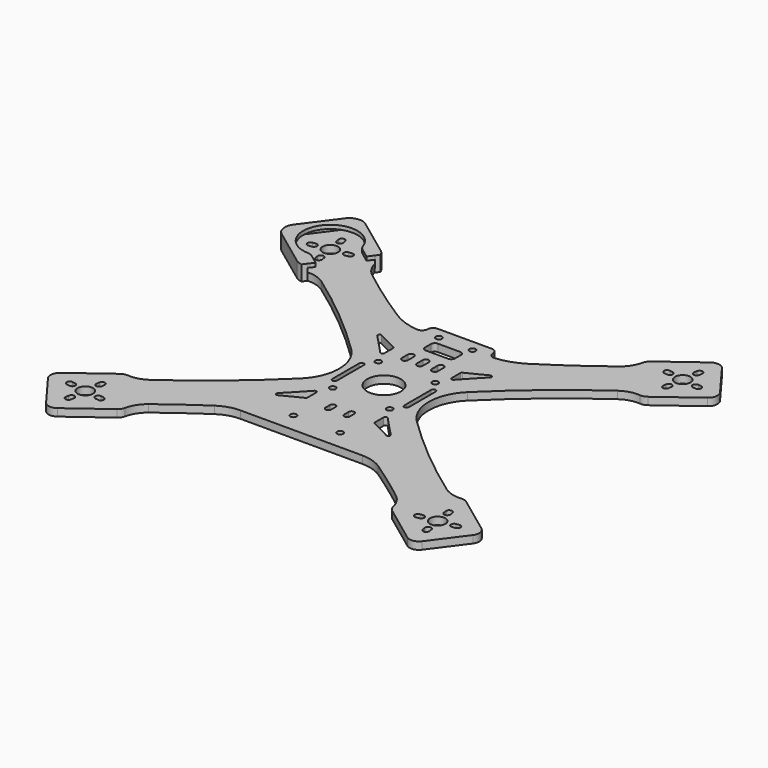
from build123d import *

# Parameters (mm, degrees)
F0_R      = 4.125
F0_R_2    = 1.625
F1_DEPTH  = 4
F3_DEPTH  = 25
F5_DEPTH  = 25
F6_R      = 9
F7_DEPTH  = 25
F8_R      = 3
F10_DEPTH = 25
F12_DEPTH = 8.1
F13_START = 2
F13_DEPTH = 4.1
F15_START = 5
F15_DEPTH = 5
F16_R     = 13
F17_DEPTH = 25


with BuildPart() as f1:
    # F0 (on Top) → F1 (new body)
    with BuildSketch(Plane.XY):
        with BuildLine():
            Line((-100.6321728581, 100.3756166522), (-113.7425143861, 82.7087282725))
            ThreePointArc((-113.7425143861, 82.7087282725), (-114.6734006575, 78.9968403849), (-112.7069355562, 75.7139032935))
            Line((-112.7069355562, 75.7139032935), (-92.6704812737, 60.8451412903))
            ThreePointArc((-92.6704812737, 60.8451412903), (-91.0578143808, 60.0508285833), (-89.2684477777, 59.8782182027))
            ThreePointArc((-89.2684477777, 59.8782182027), (-84.0566311488, 59.4038937484), (-79.3249672671, 57.1679659385))
            ThreePointArc((-79.3249672671, 57.1679659385), (-54.451545195, 38.0227925286), (-31.1542479846, 16.9880419203))
            ThreePointArc((-31.1542479846, 16.9880419203), (-24, 0), (-31.1542479846, -16.9880419203))
            ThreePointArc((-31.1542479846, -16.9880419203), (-54.451545195, -38.0227925286), (-79.3249672671, -57.1679659385))
            ThreePointArc((-79.3249672671, -57.1679659385), (-84.0566311488, -59.4038937484), (-89.2684477777, -59.8782182027))
            ThreePointArc((-89.2684477777, -59.8782182027), (-91.0578143808, -60.0508285833), (-92.6704812737, -60.8451412903))
            Line((-92.6704812737, -60.8451412903), (-112.7069355562, -75.7139032935))
            ThreePointArc((-112.7069355562, -75.7139032935), (-114.6734006575, -78.9968403849), (-113.7425143861, -82.7087282725))
            Line((-113.7425143861, -82.7087282725), (-100.6321728581, -100.3756166522))
            ThreePointArc((-100.6321728581, -100.3756166522), (-97.3492357667, -102.3420817535), (-93.6373478791, -101.4111954821))
            Line((-93.6373478791, -101.4111954821), (-73.6008935965, -86.5424334789))
            ThreePointArc((-73.6008935965, -86.5424334789), (-72.3733879407, -85.229095347), (-71.6897171476, -83.5665005586))
            ThreePointArc((-71.6897171476, -83.5665005586), (-69.7256278453, -78.7156893405), (-66.2146257391, -74.8348543181))
            ThreePointArc((-66.2146257391, -74.8348543181), (-55.1443985805, -66.5447330976), (-43.7944655315, -58.6418817782))
            ThreePointArc((-43.7944655315, -58.6418817782), (-38.4752742537, -56.1167519167), (-32.651287837, -55.25))
            Line((-32.651287837, -55.25), (32.651287837, -55.25))
            ThreePointArc((32.651287837, -55.25), (38.4752742537, -56.1167519167), (43.7944655315, -58.6418817782))
            ThreePointArc((43.7944655315, -58.6418817782), (55.1443985805, -66.5447330976), (66.2146257391, -74.8348543181))
            ThreePointArc((66.2146257391, -74.8348543181), (69.7256278453, -78.7156893405), (71.6897171476, -83.5665005586))
            ThreePointArc((71.6897171476, -83.5665005586), (72.3733879407, -85.229095347), (73.6008935965, -86.5424334789))
            Line((73.6008935965, -86.5424334789), (93.6373478791, -101.4111954821))
            ThreePointArc((93.6373478791, -101.4111954821), (97.3492357667, -102.3420817535), (100.6321728581, -100.3756166522))
            Line((100.6321728581, -100.3756166522), (113.7425143861, -82.7087282725))
            ThreePointArc((113.7425143861, -82.7087282725), (114.6734006575, -78.9968403849), (112.7069355562, -75.7139032935))
            Line((112.7069355562, -75.7139032935), (92.6704812737, -60.8451412903))
            ThreePointArc((92.6704812737, -60.8451412903), (91.0578143808, -60.0508285833), (89.2684477777, -59.8782182027))
            ThreePointArc((89.2684477777, -59.8782182027), (84.0566311488, -59.4038937484), (79.3249672671, -57.1679659385))
            ThreePointArc((79.3249672671, -57.1679659385), (54.451545195, -38.0227925286), (31.1542479846, -16.9880419203))
            ThreePointArc((31.1542479846, -16.9880419203), (24, 0), (31.1542479846, 16.9880419203))
            ThreePointArc((31.1542479846, 16.9880419203), (54.451545195, 38.0227925286), (79.3249672671, 57.1679659385))
            ThreePointArc((79.3249672671, 57.1679659385), (84.0566311488, 59.4038937484), (89.2684477777, 59.8782182027))
            ThreePointArc((89.2684477777, 59.8782182027), (91.0578143808, 60.0508285833), (92.6704812737, 60.8451412903))
            Line((92.6704812737, 60.8451412903), (112.7069355562, 75.7139032935))
            ThreePointArc((112.7069355562, 75.7139032935), (114.6734006575, 78.9968403849), (113.7425143861, 82.7087282725))
            Line((113.7425143861, 82.7087282725), (100.6321728581, 100.3756166522))
            ThreePointArc((100.6321728581, 100.3756166522), (97.3492357667, 102.3420817535), (93.6373478791, 101.4111954821))
            Line((93.6373478791, 101.4111954821), (73.6008935965, 86.5424334789))
            ThreePointArc((73.6008935965, 86.5424334789), (72.3733879407, 85.229095347), (71.6897171476, 83.5665005586))
            ThreePointArc((71.6897171476, 83.5665005586), (69.7256278453, 78.7156893405), (66.2146257391, 74.8348543181))
            ThreePointArc((66.2146257391, 74.8348543181), (50.8276984936, 63.4702586312), (34.9155456792, 52.8535285321))
            ThreePointArc((34.9155456792, 52.8535285321), (28.1194648937, 49.62008029), (20.7483484329, 48.1006910376))
            ThreePointArc((20.7483484329, 48.1006910376), (18.4683806088, 48.8830147391), (17.5, 51.090393875))
            Line((17.5, 51.090393875), (17.5, 54))
            Line((17.5, 54), (0, 54))
            Line((0, 54), (-17.5, 54))
            Line((-17.5, 54), (-17.5, 51.090393875))
            ThreePointArc((-17.5, 51.090393875), (-18.4683806088, 48.8830147391), (-20.7483484329, 48.1006910376))
            ThreePointArc((-20.7483484329, 48.1006910376), (-28.1194648937, 49.62008029), (-34.9155456792, 52.8535285321))
            ThreePointArc((-34.9155456792, 52.8535285321), (-50.8276984936, 63.4702586312), (-66.2146257391, 74.8348543181))
            ThreePointArc((-66.2146257391, 74.8348543181), (-69.7256278453, 78.7156893405), (-71.6897171476, 83.5665005586))
            ThreePointArc((-71.6897171476, 83.5665005586), (-72.3733879407, 85.229095347), (-73.6008935965, 86.5424334789))
            Line((-73.6008935965, 86.5424334789), (-93.6373478791, 101.4111954821))
            ThreePointArc((-93.6373478791, 101.4111954821), (-97.3492357667, 102.3420817535), (-100.6321728581, 100.3756166522))
        make_face()
        with Locations((-94.3386975278, -82.0073786238)):
            Circle(F0_R, mode=Mode.SUBTRACT)
        with Locations((-12.5, -45)):
            Circle(F0_R_2, mode=Mode.SUBTRACT)
        with Locations((-15.25, -15.25)):
            Circle(F0_R_2, mode=Mode.SUBTRACT)
        with Locations((94.3386975278, -82.0073786238)):
            Circle(F0_R, mode=Mode.SUBTRACT)
        with Locations((12.5, -45)):
            Circle(F0_R_2, mode=Mode.SUBTRACT)
        with Locations((15.25, -15.25)):
            Circle(F0_R_2, mode=Mode.SUBTRACT)
        with BuildLine():
            Line((-20.5, -9), (-20.5, 9))
            ThreePointArc((-20.5, 9), (-19.25, 10.25), (-18, 9))
            Line((-18, 9), (-18, -9))
            ThreePointArc((-18, -9), (-19.25, -10.25), (-20.5, -9))
        make_face(mode=Mode.SUBTRACT)
        with Locations((-15.25, 15.25)):
            Circle(F0_R_2, mode=Mode.SUBTRACT)
        with Locations((-9, 48)):
            Circle(F0_R_2, mode=Mode.SUBTRACT)
        with Locations((-94.3386975278, 82.0073786238)):
            Circle(F0_R, mode=Mode.SUBTRACT)
        with BuildLine():
            ThreePointArc((18, 9), (19.25, 10.25), (20.5, 9))
            Line((20.5, 9), (20.5, -9))
            ThreePointArc((20.5, -9), (19.25, -10.25), (18, -9))
            Line((18, -9), (18, 9))
        make_face(mode=Mode.SUBTRACT)
        with Locations((15.25, 15.25)):
            Circle(F0_R_2, mode=Mode.SUBTRACT)
        with Locations((9, 48)):
            Circle(F0_R_2, mode=Mode.SUBTRACT)
        with Locations((94.3386975278, 82.0073786238)):
            Circle(F0_R, mode=Mode.SUBTRACT)
    extrude(amount=F1_DEPTH)

    # F2 (on face) → F3 (cut)
    with BuildSketch(Plane.XY.offset(4)):
        with BuildLine():
            ThreePointArc((-97.1104772378, 89.6336727592), (-95.2650125164, 88.2641801663), (-93.8955199235, 90.1096448877))
            Line((-93.8955199235, 90.1096448877), (-94.1298446637, 91.692393104))
            ThreePointArc((-94.1298446637, 91.692393104), (-95.9753093851, 93.0618856969), (-97.344801978, 91.2164209755))
            Line((-97.344801978, 91.2164209755), (-97.1104772378, 89.6336727592))
        make_face()
        with BuildLine():
            ThreePointArc((-101.9649916632, 79.2355989138), (-100.5954990703, 81.0810636353), (-102.4409637917, 82.4505562282))
            Line((-102.4409637917, 82.4505562282), (-104.023712008, 82.216231488))
            ThreePointArc((-104.023712008, 82.216231488), (-105.3932046009, 80.3707667666), (-103.5477398795, 79.0012741737))
            Line((-103.5477398795, 79.0012741737), (-101.9649916632, 79.2355989138))
        make_face()
        with BuildLine():
            ThreePointArc((-91.5669178179, 74.3810844884), (-93.4123825393, 75.7505770813), (-94.7818751322, 73.9051123599))
            Line((-94.7818751322, 73.9051123599), (-94.547550392, 72.3223641436))
            ThreePointArc((-94.547550392, 72.3223641436), (-92.7020856706, 70.9528715507), (-91.3325930777, 72.7983362721))
            Line((-91.3325930777, 72.7983362721), (-91.5669178179, 74.3810844884))
        make_face()
        with BuildLine():
            ThreePointArc((-86.7124033925, 84.7791583338), (-88.0818959854, 82.9336936124), (-86.236431264, 81.5642010195))
            Line((-86.236431264, 81.5642010195), (-84.6536830477, 81.7985257596))
            ThreePointArc((-84.6536830477, 81.7985257596), (-83.2841904548, 83.6439904811), (-85.1296551762, 85.013483074))
            Line((-85.1296551762, 85.013483074), (-86.7124033925, 84.7791583338))
        make_face()
        with BuildLine():
            Line((94.1298446637, 91.692393104), (93.8955199235, 90.1096448877))
            ThreePointArc((93.8955199235, 90.1096448877), (95.2650125164, 88.2641801663), (97.1104772378, 89.6336727592))
            Line((97.1104772378, 89.6336727592), (97.344801978, 91.2164209755))
            ThreePointArc((97.344801978, 91.2164209755), (95.9753093851, 93.0618856969), (94.1298446637, 91.692393104))
        make_face()
        with BuildLine():
            Line((104.023712008, 82.216231488), (102.4409637917, 82.4505562282))
            ThreePointArc((102.4409637917, 82.4505562282), (100.5954990703, 81.0810636353), (101.9649916632, 79.2355989138))
            Line((101.9649916632, 79.2355989138), (103.5477398795, 79.0012741737))
            ThreePointArc((103.5477398795, 79.0012741737), (105.3932046009, 80.3707667666), (104.023712008, 82.216231488))
        make_face()
        with BuildLine():
            ThreePointArc((86.236431264, 81.5642010195), (88.0818959854, 82.9336936124), (86.7124033925, 84.7791583338))
            Line((86.7124033925, 84.7791583338), (85.1296551762, 85.013483074))
            ThreePointArc((85.1296551762, 85.013483074), (83.2841904548, 83.6439904811), (84.6536830477, 81.7985257596))
            Line((84.6536830477, 81.7985257596), (86.236431264, 81.5642010195))
        make_face()
        with BuildLine():
            Line((94.547550392, 72.3223641436), (94.7818751322, 73.9051123599))
            ThreePointArc((94.7818751322, 73.9051123599), (93.4123825393, 75.7505770813), (91.5669178179, 74.3810844884))
            Line((91.5669178179, 74.3810844884), (91.3325930777, 72.7983362721))
            ThreePointArc((91.3325930777, 72.7983362721), (92.7020856706, 70.9528715507), (94.547550392, 72.3223641436))
        make_face()
        with BuildLine():
            Line((-94.1298446637, -91.692393104), (-93.8955199235, -90.1096448877))
            ThreePointArc((-93.8955199235, -90.1096448877), (-95.2650125164, -88.2641801663), (-97.1104772378, -89.6336727592))
            Line((-97.1104772378, -89.6336727592), (-97.344801978, -91.2164209755))
            ThreePointArc((-97.344801978, -91.2164209755), (-95.9753093851, -93.0618856969), (-94.1298446637, -91.692393104))
        make_face()
        with BuildLine():
            Line((-104.023712008, -82.216231488), (-102.4409637917, -82.4505562282))
            ThreePointArc((-102.4409637917, -82.4505562282), (-100.5954990703, -81.0810636353), (-101.9649916632, -79.2355989138))
            Line((-101.9649916632, -79.2355989138), (-103.5477398795, -79.0012741737))
            ThreePointArc((-103.5477398795, -79.0012741737), (-105.3932046009, -80.3707667666), (-104.023712008, -82.216231488))
        make_face()
        with BuildLine():
            ThreePointArc((86.7124033925, -84.7791583338), (88.0818959854, -82.9336936124), (86.236431264, -81.5642010195))
            Line((86.236431264, -81.5642010195), (84.6536830477, -81.7985257596))
            ThreePointArc((84.6536830477, -81.7985257596), (83.2841904548, -83.6439904811), (85.1296551762, -85.013483074))
            Line((85.1296551762, -85.013483074), (86.7124033925, -84.7791583338))
        make_face()
        with BuildLine():
            Line((97.344801978, -91.2164209755), (97.1104772378, -89.6336727592))
            ThreePointArc((97.1104772378, -89.6336727592), (95.2650125164, -88.2641801663), (93.8955199235, -90.1096448877))
            Line((93.8955199235, -90.1096448877), (94.1298446637, -91.692393104))
            ThreePointArc((94.1298446637, -91.692393104), (95.9753093851, -93.0618856969), (97.344801978, -91.2164209755))
        make_face()
        with BuildLine():
            Line((103.5477398795, -79.0012741737), (101.9649916632, -79.2355989138))
            ThreePointArc((101.9649916632, -79.2355989138), (100.5954990703, -81.0810636353), (102.4409637917, -82.4505562282))
            Line((102.4409637917, -82.4505562282), (104.023712008, -82.216231488))
            ThreePointArc((104.023712008, -82.216231488), (105.3932046009, -80.3707667666), (103.5477398795, -79.0012741737))
        make_face()
        with BuildLine():
            Line((91.3325930777, -72.7983362721), (91.5669178179, -74.3810844884))
            ThreePointArc((91.5669178179, -74.3810844884), (93.4123825393, -75.7505770813), (94.7818751322, -73.9051123599))
            Line((94.7818751322, -73.9051123599), (94.547550392, -72.3223641436))
            ThreePointArc((94.547550392, -72.3223641436), (92.7020856706, -70.9528715507), (91.3325930777, -72.7983362721))
        make_face()
        with BuildLine():
            ThreePointArc((-94.7818751322, -73.9051123599), (-93.4123825393, -75.7505770813), (-91.5669178179, -74.3810844884))
            Line((-91.5669178179, -74.3810844884), (-91.3325930777, -72.7983362721))
            ThreePointArc((-91.3325930777, -72.7983362721), (-92.7020856706, -70.9528715507), (-94.547550392, -72.3223641436))
            Line((-94.547550392, -72.3223641436), (-94.7818751322, -73.9051123599))
        make_face()
        with BuildLine():
            Line((-86.7124033925, -84.7791583338), (-85.1296551762, -85.013483074))
            ThreePointArc((-85.1296551762, -85.013483074), (-83.2841904548, -83.6439904811), (-84.6536830477, -81.7985257596))
            Line((-84.6536830477, -81.7985257596), (-86.236431264, -81.5642010195))
            ThreePointArc((-86.236431264, -81.5642010195), (-88.0818959854, -82.9336936124), (-86.7124033925, -84.7791583338))
        make_face()
    extrude(amount=-F3_DEPTH, mode=Mode.SUBTRACT)

    # F4 (on face) → F5 (cut)
    with BuildSketch(Plane.XY.offset(4)):
        with BuildLine():
            ThreePointArc((-6.375, 28), (-8, 29.625), (-9.625, 28))
            Line((-9.625, 28), (-9.625, 24))
            ThreePointArc((-9.625, 24), (-8, 22.375), (-6.375, 24))
            Line((-6.375, 24), (-6.375, 28))
        make_face()
        with BuildLine():
            ThreePointArc((1.625, 28), (0, 29.625), (-1.625, 28))
            Line((-1.625, 28), (-1.625, 24))
            ThreePointArc((-1.625, 24), (0, 22.375), (1.625, 24))
            Line((1.625, 24), (1.625, 28))
        make_face()
        with BuildLine():
            ThreePointArc((9.625, 28), (8, 29.625), (6.375, 28))
            Line((6.375, 28), (6.375, 24))
            ThreePointArc((6.375, 24), (8, 22.375), (9.625, 24))
            Line((9.625, 24), (9.625, 28))
        make_face()
    extrude(amount=-F5_DEPTH, mode=Mode.SUBTRACT)

    # F6 (on face) → F7 (cut)
    with BuildSketch(Plane.XY.offset(4)):
        with BuildLine():
            Line((6, 43.5), (-6, 43.5))
            ThreePointArc((-6, 43.5), (-7.4142135624, 42.9142135624), (-8, 41.5))
            Line((-8, 41.5), (-8, 37.5))
            ThreePointArc((-8, 37.5), (-7.4142135624, 36.0857864376), (-6, 35.5))
            Line((-6, 35.5), (6, 35.5))
            ThreePointArc((6, 35.5), (7.4142135624, 36.0857864376), (8, 37.5))
            Line((8, 37.5), (8, 41.5))
            ThreePointArc((8, 41.5), (7.4142135624, 42.9142135624), (6, 43.5))
        make_face()
        with BuildLine():
            ThreePointArc((-3.5, -28), (-5, -26.5), (-6.5, -28))
            Line((-6.5, -28), (-6.5, -31))
            ThreePointArc((-6.5, -31), (-5, -32.5), (-3.5, -31))
            Line((-3.5, -31), (-3.5, -28))
        make_face()
        with BuildLine():
            ThreePointArc((6.5, -28), (5, -26.5), (3.5, -28))
            Line((3.5, -28), (3.5, -31))
            ThreePointArc((3.5, -31), (5, -32.5), (6.5, -31))
            Line((6.5, -31), (6.5, -28))
        make_face()
        Circle(F6_R)
    extrude(amount=-F7_DEPTH, mode=Mode.SUBTRACT)

    # F8
    f8_edges = [f1.edges().sort_by_distance(p)[0] for p in [
        (-17.5, 54, 2),
        (17.5, 54, 2),
    ]]
    fillet(f8_edges, radius=F8_R)

    # F9 (on face) → F10 (cut)
    with BuildSketch(Plane.XY.offset(4)):
        with BuildLine():
            ThreePointArc((-18.5615734392, 29.4784741395), (-23.8228134976, 32.0929109704), (-29.0451265181, 34.7842626031))
            ThreePointArc((-29.0451265181, 34.7842626031), (-30.3127764029, 34.494671544), (-30.2226462445, 33.1974916156))
            ThreePointArc((-30.2226462445, 33.1974916156), (-24.9281613816, 27.7115010311), (-19.7390931656, 22.1256945802))
            ThreePointArc((-19.7390931656, 22.1256945802), (-18.6388166433, 21.8668029796), (-18, 22.7992977961))
            Line((-18, 22.7992977961), (-18, 28.5797071226))
            ThreePointArc((-18, 28.5797071226), (-18.1519355682, 29.1096002435), (-18.5615734392, 29.4784741395))
        make_face()
        with BuildLine():
            ThreePointArc((18.5615734392, 29.4784741395), (18.1519355682, 29.1096002435), (18, 28.5797071226))
            Line((18, 28.5797071226), (18, 22.7992977961))
            ThreePointArc((18, 22.7992977961), (18.6388166433, 21.8668029796), (19.7390931656, 22.1256945802))
            ThreePointArc((19.7390931656, 22.1256945802), (24.9281613816, 27.7115010311), (30.2226462445, 33.1974916156))
            ThreePointArc((30.2226462445, 33.1974916156), (30.3127764029, 34.494671544), (29.0451265181, 34.7842626031))
            ThreePointArc((29.0451265181, 34.7842626031), (23.8228134976, 32.0929109704), (18.5615734392, 29.4784741395))
        make_face()
        with BuildLine():
            Line((18, -22.7992977961), (18, -28.5797071226))
            ThreePointArc((18, -28.5797071226), (18.1519355682, -29.1096002435), (18.5615734392, -29.4784741395))
            ThreePointArc((18.5615734392, -29.4784741395), (23.8228134976, -32.0929109704), (29.0451265181, -34.7842626031))
            ThreePointArc((29.0451265181, -34.7842626031), (30.3127764029, -34.494671544), (30.2226462445, -33.1974916156))
            ThreePointArc((30.2226462445, -33.1974916156), (24.9281613816, -27.7115010311), (19.7390931656, -22.1256945802))
            ThreePointArc((19.7390931656, -22.1256945802), (18.6388166433, -21.8668029796), (18, -22.7992977961))
        make_face()
        with BuildLine():
            ThreePointArc((-18.5615734392, -29.4784741395), (-18.1519355682, -29.1096002435), (-18, -28.5797071226))
            Line((-18, -28.5797071226), (-18, -22.7992977961))
            ThreePointArc((-18, -22.7992977961), (-18.6388166433, -21.8668029796), (-19.7390931656, -22.1256945802))
            ThreePointArc((-19.7390931656, -22.1256945802), (-24.9281613816, -27.7115010311), (-30.2226462445, -33.1974916156))
            ThreePointArc((-30.2226462445, -33.1974916156), (-30.3127764029, -34.494671544), (-29.0451265181, -34.7842626031))
            ThreePointArc((-29.0451265181, -34.7842626031), (-23.8228134976, -32.0929109704), (-18.5615734392, -29.4784741395))
        make_face()
    extrude(amount=-F10_DEPTH, mode=Mode.SUBTRACT)


with BuildPart() as f12:
    # F11 (on Top) → F12 (new body)
    with BuildSketch(Plane.XY):
        with BuildLine():
            ThreePointArc((-88.8877311806, 59.8189111944), (-90.8824777053, 59.8898839037), (-92.6905184954, 60.7354838827))
            Line((-92.6905184954, 60.7354838827), (-112.8468320558, 75.6931917169))
            ThreePointArc((-112.8468320558, 75.6931917169), (-114.8132971571, 78.9761288083), (-113.8824108857, 82.688016696))
            Line((-113.8824108857, 82.688016696), (-100.6528844347, 100.5155131518))
            ThreePointArc((-100.6528844347, 100.5155131518), (-97.3699473433, 102.4819782531), (-93.6580594557, 101.5510919817))
            Line((-93.6580594557, 101.5510919817), (-73.5017458953, 86.5933841474))
            ThreePointArc((-73.5017458953, 86.5933841474), (-72.1685438957, 85.1079134303), (-71.5226424676, 83.2192996084))
            Line((-71.5226424676, 83.2192996084), (-70.0128900453, 85.2537719728))
            ThreePointArc((-70.0128900453, 85.2537719728), (-70.9612768277, 86.8826662704), (-72.3098966655, 88.1994649092))
            Line((-72.3098966655, 88.1994649092), (-92.4662102259, 103.1571727435))
            ThreePointArc((-92.4662102259, 103.1571727435), (-97.6628532686, 104.4604135234), (-102.2589651965, 101.7073623816))
            Line((-102.2589651965, 101.7073623816), (-115.4884916475, 83.8798659258))
            ThreePointArc((-115.4884916475, 83.8798659258), (-116.7917324275, 78.6832228831), (-114.0386812856, 74.0871109552))
            Line((-114.0386812856, 74.0871109552), (-93.8823677252, 59.1294031209))
            ThreePointArc((-93.8823677252, 59.1294031209), (-92.2312962141, 58.2201743339), (-90.397483603, 57.78443883))
            Line((-90.397483603, 57.78443883), (-88.8877311806, 59.8189111944))
        make_face()
        with BuildLine():
            Line((-112.8468320558, 75.6931917169), (-92.6905184954, 60.7354838827))
            ThreePointArc((-92.6905184954, 60.7354838827), (-90.8824777053, 59.8898839037), (-88.8877311806, 59.8189111944))
            Line((-88.8877311806, 59.8189111944), (-71.5226424676, 83.2192996084))
            ThreePointArc((-71.5226424676, 83.2192996084), (-72.1685438957, 85.1079134303), (-73.5017458953, 86.5933841474))
            Line((-73.5017458953, 86.5933841474), (-93.6580594557, 101.5510919817))
            ThreePointArc((-93.6580594557, 101.5510919817), (-97.3699473433, 102.4819782531), (-100.6528844347, 100.5155131518))
            Line((-100.6528844347, 100.5155131518), (-113.8824108857, 82.688016696))
            ThreePointArc((-113.8824108857, 82.688016696), (-114.8132971571, 78.9761288083), (-112.8468320558, 75.6931917169))
        make_face()
    extrude(amount=F12_DEPTH)

    # F11 (on Top) → F13 (cut)
    with BuildSketch(Plane.XY.offset(F13_START)):
        with BuildLine():
            Line((-112.8468320558, 75.6931917169), (-92.6905184954, 60.7354838827))
            ThreePointArc((-92.6905184954, 60.7354838827), (-90.8824777053, 59.8898839037), (-88.8877311806, 59.8189111944))
            Line((-88.8877311806, 59.8189111944), (-71.5226424676, 83.2192996084))
            ThreePointArc((-71.5226424676, 83.2192996084), (-72.1685438957, 85.1079134303), (-73.5017458953, 86.5933841474))
            Line((-73.5017458953, 86.5933841474), (-93.6580594557, 101.5510919817))
            ThreePointArc((-93.6580594557, 101.5510919817), (-97.3699473433, 102.4819782531), (-100.6528844347, 100.5155131518))
            Line((-100.6528844347, 100.5155131518), (-113.8824108857, 82.688016696))
            ThreePointArc((-113.8824108857, 82.688016696), (-114.8132971571, 78.9761288083), (-112.8468320558, 75.6931917169))
        make_face()
    extrude(amount=F13_DEPTH, mode=Mode.SUBTRACT)

    # F14 (on face) → F15 (cut)
    with BuildSketch(Plane.XY.offset(F15_START)):
        with BuildLine():
            ThreePointArc((-78.8322376791, 84.198201063), (-79.8982377297, 85.2752175531), (-80.592635867, 86.6221146742))
            ThreePointArc((-80.592635867, 86.6221146742), (-105.9827830508, 90.64828554), (-94.7725856781, 67.5138717648))
            ThreePointArc((-94.7725856781, 67.5138717648), (-93.2822660549, 67.2395215351), (-91.9425792071, 66.5313126834))
            Line((-91.9425792071, 66.5313126834), (-86.7603575881, 62.6856612116))
            Line((-86.7603575881, 62.6856612116), (-73.6500160601, 80.3525495912))
            Line((-73.6500160601, 80.3525495912), (-78.8322376791, 84.198201063))
        make_face()
    extrude(amount=F15_DEPTH, mode=Mode.SUBTRACT)

    # F16 (on face) → F17 (cut)
    with BuildSketch(Plane(origin=(0, 0, 0), x_dir=(1, 0, 0), z_dir=(0, 0, -1))):
        with Locations((-94.5394576231, -82.1563597775)):
            Circle(F16_R)
    extrude(amount=-F17_DEPTH, mode=Mode.SUBTRACT)


solid = Compound([f1.part, f12.part])
